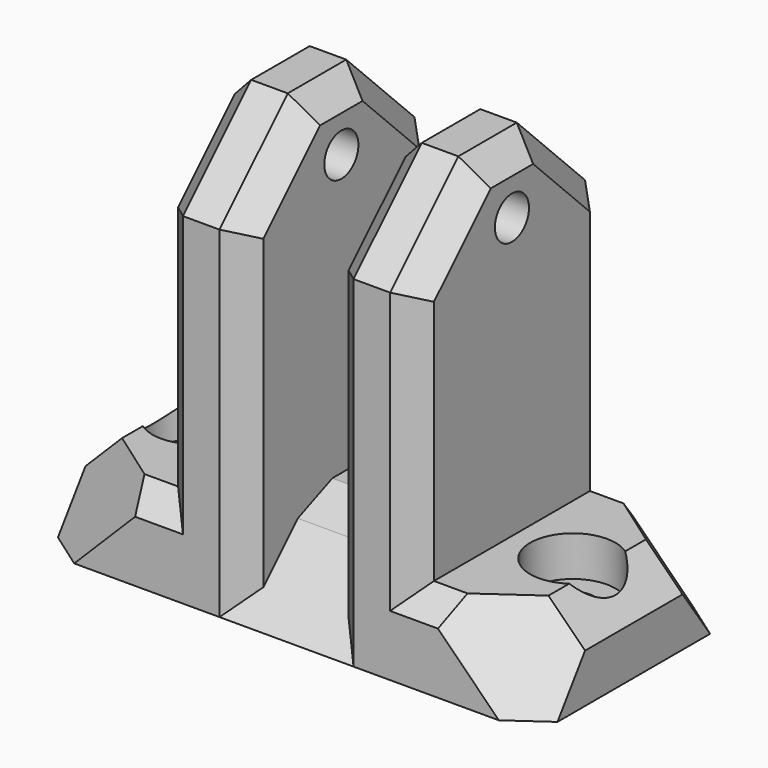
from build123d import *

# Parameters (mm, degrees)
F0_W          = 10
F0_H          = 7
F0_W_2        = 7
F0_H_2        = 28
F1_DEPTH      = 20
F2_R          = 3.5
F2_R_2        = 1.75
F3_DEPTH      = 3.3
F4_DEPTH      = 25
F6_DEPTH      = 3.3
F7_DEPTH      = 25
F9_DEPTH      = 25
F10_SIZE      = 7
F11_T1_DEPTH  = 35.4300979278
F12_SIZE      = 6.99999
F13_T1_DEPTH  = 7
F13_T6_DEPTH  = 29.9594705668
F13_T11_DEPTH = 29.9594705668
F13_T16_DEPTH = 29.9594705668
F13_T21_DEPTH = 29.9594705668
F14_T1_DEPTH  = 26.1433659759
F14_T3_DEPTH  = 20.1862268885
F14_T5_DEPTH  = 20.1862268885
F14_T10_DEPTH = 38.2867219519
F14_T15_DEPTH = 38.2867219519
F14_T20_DEPTH = 38.2867219519
F14_T25_DEPTH = 38.2867219519
F15_SIZE      = 2
F16_SIZE      = 2


# Not quite as in the source:
# - a fillet or chamfer that OpenCascade refuses, or shapes differently, is made with other operations: its cross-section is extruded or revolved along the edge and cut away or added
# - a fillet or chamfer is up to 0.001 mm smaller than in the source, because OpenCascade refuses the exact size


with BuildPart() as f1:
    # F0 (on Front) → F1 (new body)
    with BuildSketch(Plane.XZ):
        with Locations((-15.5, 3.5)):
            Rectangle(F0_W, F0_H)
        with Locations((-7, 3.5)):
            Rectangle(F0_W_2, F0_H)
        with Locations((0, 3.5)):
            Rectangle(F0_W_2, F0_H)
        with Locations((-7, 21)):
            Rectangle(F0_W_2, F0_H_2)
        with Locations((7, 3.5)):
            Rectangle(F0_W_2, F0_H)
        with Locations((15.5, 3.5)):
            Rectangle(F0_W, F0_H)
        with Locations((7, 21)):
            Rectangle(F0_W_2, F0_H_2)
    extrude(amount=F1_DEPTH)

    # F2 (on face) → F3 (cut)
    with BuildSketch(Plane.XY.offset(7)):
        with Locations((15.5, -10)):
            Circle(F2_R)
        with Locations((15.5, -10)):
            Circle(F2_R_2, mode=Mode.SUBTRACT)
    extrude(amount=-F3_DEPTH, mode=Mode.SUBTRACT)

    # F2 (on face) → F4 (cut)
    with BuildSketch(Plane.XY.offset(7)):
        with Locations((15.5, -10)):
            Circle(F2_R_2)
    extrude(amount=-F4_DEPTH, mode=Mode.SUBTRACT)

    # F5 (on face) → F6 (cut)
    with BuildSketch(Plane.XY.offset(7)):
        with BuildLine():
            ThreePointArc((-12, -10), (-15.5, -6.5), (-19, -10))
            ThreePointArc((-19, -10), (-15.5, -13.5), (-12, -10))
        make_face()
        with BuildLine():
            ThreePointArc((-13.75, -10), (-15.5, -11.75), (-17.25, -10))
            ThreePointArc((-17.25, -10), (-15.5, -8.25), (-13.75, -10))
        make_face(mode=Mode.SUBTRACT)
    extrude(amount=-F6_DEPTH, mode=Mode.SUBTRACT)

    # F7 (cut): a face of the model
    f7_faces = [f1.faces().sort_by_distance(p)[0] for p in [
        (-15.5, -10, 7),
    ]]
    extrude(f7_faces, amount=-F7_DEPTH, mode=Mode.SUBTRACT)

    # F8 (on face) → F9 (cut)
    with BuildSketch(Plane(origin=(-10.5, 0, 0), x_dir=(0, -1, 0), z_dir=(-1, 0, 0))):
        with BuildLine():
            ThreePointArc((10, 31.75), (8.7625631329, 28.7625631329), (11.75, 30))
            ThreePointArc((11.75, 30), (11.2374368671, 31.2374368671), (10, 31.75))
        make_face()
    extrude(amount=-F9_DEPTH, mode=Mode.SUBTRACT)

    # F10
    f10_edges = [f1.edges().sort_by_distance(p)[0] for p in [
        (-7, -20, 35),
        (-7, 0, 35),
        (7, 0, 35),
        (7, -20, 35),
    ]]
    chamfer(f10_edges, length=F10_SIZE)

    # F11: chamfer of 3 on 2 edges, made by hand

    # F11_s2 → F11_t1 (cut)
    with BuildSketch(Plane.XZ.offset(-7.7150489639)):
        Polygon((17.5, 7), (20.5, 4), (20.5, 7), align=None)
        Polygon((-20.5, 4), (-17.5, 7), (-20.5, 7), align=None)
    extrude(amount=F11_T1_DEPTH, mode=Mode.SUBTRACT)

    # F12 (size 7 in the source; OpenCascade refuses exactly that, so slightly less here)
    f12_edges = [f1.edges().sort_by_distance(p)[0] for p in [
        (0, 0, 7),
        (0, -20, 7),
    ]]
    chamfer(f12_edges, length=F12_SIZE)

    # F13: chamfer of 5 on 6 edges, made by hand

    # F13_s2 → F13_t1 (cut)
    with BuildSketch(Plane.YZ.offset(-3.5)):
        Polygon((-5.5355239059, 5.5355339059), (-9.0710578119, 7), (-6.99999, 7), align=None)
        Polygon((-10.9289421881, 7), (-14.4644760941, 5.5355339059), (-13.00001, 7), align=None)
    extrude(amount=F13_T1_DEPTH, mode=Mode.SUBTRACT)


with BuildPart() as f13_tool4:
    # F13_s5 → F13_t6 (new body)
    with BuildSketch(Plane(origin=(17.3422723993, 0, -17.3422723993), x_dir=(0, 1, 0), z_dir=(-0.7071067812, 0, 0.7071067812))):
        Polygon((-15, -17.3241161391), (-20, -12.3241161391), (-20, -17.3241161391), align=None)
    extrude(amount=F13_T6_DEPTH)

    split(bisect_by=Plane.XY.offset(7), keep=Keep.BOTTOM)


with BuildPart() as f1_1:
    add(f1.part)

    # F13_t3: cut F13_tool4
    add(f13_tool4.part, mode=Mode.SUBTRACT)


with BuildPart() as f13_tool9:
    # F13_s10 → F13_t11 (new body)
    with BuildSketch(Plane(origin=(17.3422723993, 0, -17.3422723993), x_dir=(0, 1, 0), z_dir=(-0.7071067812, 0, 0.7071067812))):
        Polygon((0, -12.3241161391), (-5, -17.3241161391), (0, -17.3241161391), align=None)
    extrude(amount=F13_T11_DEPTH)

    split(bisect_by=Plane.XY.offset(7), keep=Keep.BOTTOM)


with BuildPart() as f1_2:
    add(f1_1.part)

    # F13_t8: cut F13_tool9
    add(f13_tool9.part, mode=Mode.SUBTRACT)


with BuildPart() as f13_tool14:
    # F13_s15 → F13_t16 (new body)
    with BuildSketch(Plane(origin=(3.8422723993, 0, 3.8422723993), x_dir=(0, 1, 0), z_dir=(-0.7071067812, 0, -0.7071067812))):
        Polygon((0, -12.3241161391), (-5, -17.3241161391), (0, -17.3241161391), align=None)
    extrude(amount=F13_T16_DEPTH)

    split(bisect_by=Plane.XY.offset(7), keep=Keep.BOTTOM)


with BuildPart() as f1_3:
    add(f1_2.part)

    # F13_t13: cut F13_tool14
    add(f13_tool14.part, mode=Mode.SUBTRACT)


with BuildPart() as f13_tool19:
    # F13_s20 → F13_t21 (new body)
    with BuildSketch(Plane(origin=(3.8422723993, 0, 3.8422723993), x_dir=(0, 1, 0), z_dir=(-0.7071067812, 0, -0.7071067812))):
        Polygon((-15, -17.3241161391), (-20, -12.3241161391), (-20, -17.3241161391), align=None)
    extrude(amount=F13_T21_DEPTH)

    split(bisect_by=Plane.XY.offset(7), keep=Keep.BOTTOM)


with BuildPart() as f1_4:
    add(f1_3.part)

    # F13_t18: cut F13_tool19
    add(f13_tool19.part, mode=Mode.SUBTRACT)

    # F14: chamfer of 2 on 16 edges, made by hand

    # F14_s2 → F14_t1 (cut)
    with BuildSketch(Plane.XY.offset(7)):
        Polygon((-10.5, -18), (-8.5, -20), (-10.5, -20), align=None)
        Polygon((10.5, -18), (8.5, -20), (10.5, -20), align=None)
        Polygon((8.5, 0), (10.5, -2), (10.5, 0), align=None)
        Polygon((-8.5, 0), (-10.5, -2), (-10.5, 0), align=None)
    extrude(amount=F14_T1_DEPTH, mode=Mode.SUBTRACT)

    # F14_s4 → F14_t3 (cut)
    with BuildSketch(Plane(origin=(0, 0.3630910403, 0.3630910403), x_dir=(1, 0, 0), z_dir=(0, 0.7071067812, 0.7071067812))):
        Polygon((10.5, -31.941125497), (8.5, -33.941125497), (10.5, -33.941125497), align=None)
        Polygon((3.5, -31.941125497), (5.5, -33.941125497), (3.5, -33.941125497), align=None)
        Polygon((-10.5, -31.941125497), (-8.5, -33.941125497), (-10.5, -33.941125497), align=None)
        Polygon((-3.5, -31.941125497), (-5.5, -33.941125497), (-3.5, -33.941125497), align=None)
    extrude(amount=F14_T3_DEPTH, mode=Mode.SUBTRACT)

    # F14_s6 → F14_t5 (cut)
    with BuildSketch(Plane(origin=(0, -10.3630910403, 10.3630910403), x_dir=(1, 0, 0), z_dir=(0, -0.7071067812, 0.7071067812))):
        Polygon((3.5, 17.7989898732), (5.5, 19.7989898732), (3.5, 19.7989898732), align=None)
        Polygon((8.5, 19.7989898732), (10.5, 17.7989898732), (10.5, 19.7989898732), align=None)
        Polygon((-5.5, 19.7989898732), (-3.5, 17.7989898732), (-3.5, 19.7989898732), align=None)
        Polygon((-10.5, 17.7989898732), (-8.5, 19.7989898732), (-10.5, 19.7989898732), align=None)
    extrude(amount=F14_T5_DEPTH, mode=Mode.SUBTRACT)


with BuildPart() as f14_tool8:
    # F14_s9 → F14_t10 (new body)
    with BuildSketch(Plane.XY.offset(33.1433659759)):
        Polygon((-3.5, -18), (-5.5, -20), (-3.5, -20), align=None)
    extrude(amount=-F14_T10_DEPTH)

    split(bisect_by=Plane(origin=(0, -10.000005, 10.000005), x_dir=(1, 0, 0), z_dir=(0, -0.7071067812, 0.7071067812)), keep=Keep.TOP)


with BuildPart() as f1_5:
    add(f1_4.part)

    # F14_t7: cut F14_tool8
    add(f14_tool8.part, mode=Mode.SUBTRACT)


with BuildPart() as f14_tool13:
    # F14_s14 → F14_t15 (new body)
    with BuildSketch(Plane.XY.offset(-5.1433559759)):
        Polygon((3.5, -18), (5.5, -20), (3.5, -20), align=None)
    extrude(amount=F14_T15_DEPTH)

    split(bisect_by=Plane(origin=(0, -10.000005, 10.000005), x_dir=(1, 0, 0), z_dir=(0, -0.7071067812, 0.7071067812)), keep=Keep.TOP)


with BuildPart() as f1_6:
    add(f1_5.part)

    # F14_t12: cut F14_tool13
    add(f14_tool13.part, mode=Mode.SUBTRACT)


with BuildPart() as f14_tool18:
    # F14_s19 → F14_t20 (new body)
    with BuildSketch(Plane.XY.offset(-5.1433559759)):
        Polygon((5.5, 0), (3.5, -2), (3.5, 0), align=None)
    extrude(amount=F14_T20_DEPTH)

    split(bisect_by=Plane(origin=(0, 5e-06, 5e-06), x_dir=(1, 0, 0), z_dir=(0, 0.7071067812, 0.7071067812)), keep=Keep.TOP)


with BuildPart() as f1_7:
    add(f1_6.part)

    # F14_t17: cut F14_tool18
    add(f14_tool18.part, mode=Mode.SUBTRACT)


with BuildPart() as f14_tool23:
    # F14_s24 → F14_t25 (new body)
    with BuildSketch(Plane.XY.offset(33.1433659759)):
        Polygon((-5.5, 0), (-3.5, -2), (-3.5, 0), align=None)
    extrude(amount=-F14_T25_DEPTH)

    split(bisect_by=Plane(origin=(0, 5e-06, 5e-06), x_dir=(1, 0, 0), z_dir=(0, 0.7071067812, 0.7071067812)), keep=Keep.TOP)


with BuildPart() as f1_8:
    add(f1_7.part)

    # F14_t22: cut F14_tool23
    add(f14_tool23.part, mode=Mode.SUBTRACT)

    # F15
    f15_edges = [f1_8.edges().sort_by_distance(p)[0] for p in [
        (10.5, -10, 35),
        (3.5, -10, 35),
        (-3.5, -10, 35),
        (-10.5, -10, 35),
    ]]
    chamfer(f15_edges, length=F15_SIZE)

    # F16
    f16_edges = [f1_8.edges().sort_by_distance(p)[0] for p in [
        (-9.464466, 0, 7),
        (9.464466, 0, 7),
        (-9.464466, -20, 7),
        (9.464466, -20, 7),
    ]]
    chamfer(f16_edges, length=F16_SIZE)


solid = f1_8.part
